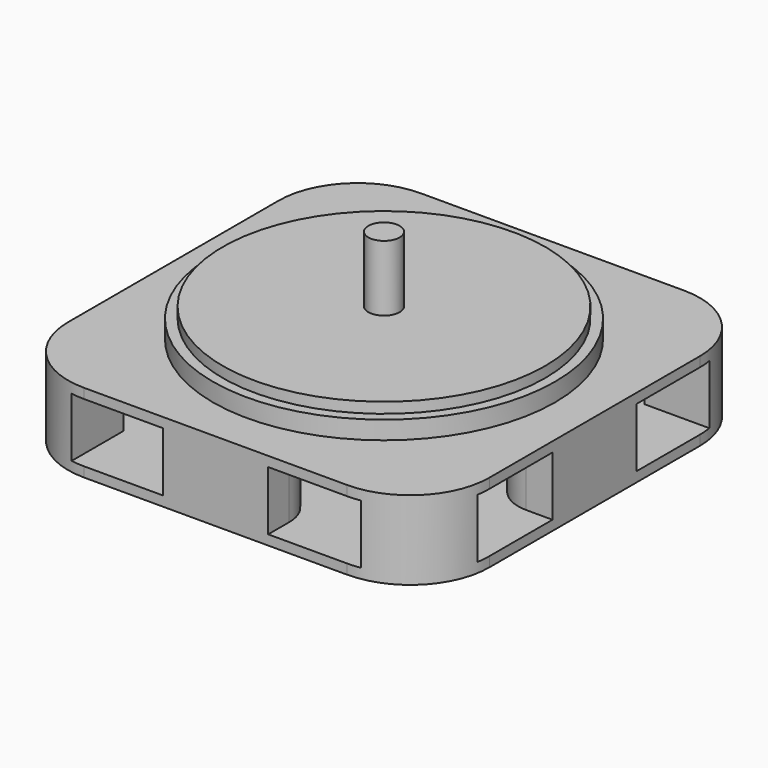
from build123d import *

# Parameters (mm, degrees)
F0_R         = 311.15
F1_DEPTH     = 20.574
F2_R         = 330.2
F3_DEPTH     = 35.052
F4_W         = 812.8
F4_H         = 812.8
F5_DEPTH     = 152.4
F6_W         = 177.8
F6_H         = 114.3
F7_DEPTH     = 812.801
F8_W         = 177.8
F8_H         = 114.3
F9_DEPTH     = 812.801
F10_T1_DEPTH = 914.4
F11_R        = 76.2
F12_R        = 30.1625
F13_DEPTH    = 127


# Not quite as in the source:
# - a fillet or chamfer that OpenCascade refuses, or shapes differently, is made with other operations: its cross-section is extruded or revolved along the edge and cut away or added


with BuildPart() as f1:
    # F0 (on Top) → F1 (new body)
    with BuildSketch(Plane.XY):
        Circle(F0_R)
    extrude(amount=F1_DEPTH)

    # F2 (on face) → F3 (join)
    with BuildSketch(Plane(origin=(0, 0, 0), x_dir=(1, 0, 0), z_dir=(0, 0, -1))):
        Circle(F2_R)
    extrude(amount=F3_DEPTH)

    # F4 (on face) → F5 (join)
    with BuildSketch(Plane(origin=(0, 0, -35.052), x_dir=(1, 0, 0), z_dir=(0, 0, -1))):
        Rectangle(F4_W, F4_H)
    extrude(amount=F5_DEPTH)

    # F6 (on face) → F7 (cut, through all)
    with BuildSketch(Plane(origin=(0, 406.4, 0), x_dir=(-1, 0, 0), z_dir=(0, 1, 0))):
        with Locations((190.5, -111.252)):
            Rectangle(F6_W, F6_H)
        with Locations((-190.5, -111.252)):
            Rectangle(F6_W, F6_H)
    extrude(amount=-F7_DEPTH, mode=Mode.SUBTRACT)

    # F8 (on face) → F9 (cut, through all)
    with BuildSketch(Plane(origin=(-406.4, 0, 0), x_dir=(0, -1, 0), z_dir=(-1, 0, 0))):
        with Locations((190.5, -111.252)):
            Rectangle(F8_W, F8_H)
        with Locations((-190.5, -111.252)):
            Rectangle(F8_W, F8_H)
    extrude(amount=-F9_DEPTH, mode=Mode.SUBTRACT)

    # F10: fillet of radius 152.4 on 4 edges, made by hand

    # F10_s2 → F10_t1 (cut)
    with BuildSketch(Plane.XY.offset(-568.452)):
        with BuildLine():
            ThreePointArc((-254, -406.4), (-361.7630734528, -361.7630734528), (-406.4, -254))
            Line((-406.4, -254), (-406.4, -406.4))
            Line((-406.4, -406.4), (-254, -406.4))
        make_face()
        with BuildLine():
            ThreePointArc((-254, 406.4), (-361.7630734528, 361.7630734528), (-406.4, 254))
            Line((-406.4, 254), (-406.4, 406.4))
            Line((-406.4, 406.4), (-254, 406.4))
        make_face()
        with BuildLine():
            ThreePointArc((406.4, 254), (361.7630734528, 361.7630734528), (254, 406.4))
            Line((254, 406.4), (406.4, 406.4))
            Line((406.4, 406.4), (406.4, 254))
        make_face()
        with BuildLine():
            ThreePointArc((406.4, -254), (361.7630734528, -361.7630734528), (254, -406.4))
            Line((254, -406.4), (406.4, -406.4))
            Line((406.4, -406.4), (406.4, -254))
        make_face()
    extrude(amount=F10_T1_DEPTH, mode=Mode.SUBTRACT)

    # F11
    f11_edges = [f1.edges().sort_by_distance(p)[0] for p in [
        (279.4, -101.6, -111.252),
        (279.4, 101.6, -111.252),
        (101.6, 279.4, -111.252),
        (-101.6, 279.4, -111.252),
        (-279.4, 101.6, -111.252),
        (-279.4, -101.6, -111.252),
        (-101.6, -279.4, -111.252),
        (101.6, -279.4, -111.252),
    ]]
    fillet(f11_edges, radius=F11_R)

    # F12 (on face) → F13 (join)
    with BuildSketch(Plane.XY.offset(20.574)):
        Circle(F12_R)
    extrude(amount=F13_DEPTH)


solid = f1.part
